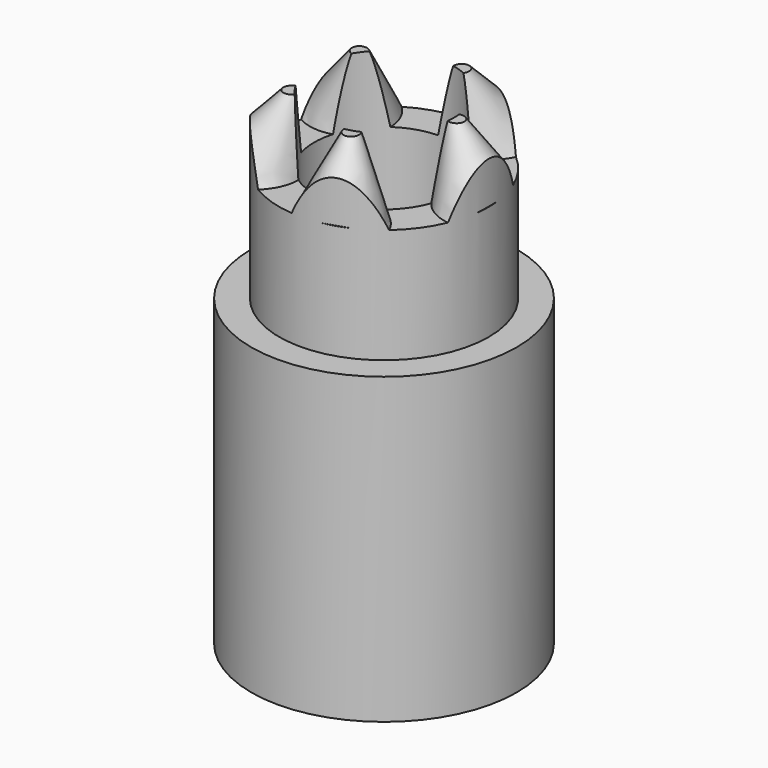
from build123d import *

# Parameters (mm, degrees)
F0_R      = 1.5
F0_R_2    = 1
F1_DEPTH  = 2.6
F5_COUNT  = 5
F5_ANGLE  = 288
F17_DEPTH = 1.64
F0_R_3    = 1.9
F18_DEPTH = 4.35


with BuildPart() as f1:
    # F0 (on Top) → F1 (new body)
    with BuildSketch(Plane.XY):
        Circle(F0_R)
        Circle(F0_R_2, mode=Mode.SUBTRACT)
    extrude(amount=F1_DEPTH)


with BuildPart() as f4:
    # F3 (on Front) → F4 (revolve)
    with BuildSketch(Plane.XZ):
        Polygon((0.9303738137, 2.820600407), (1.375, 1.599), (1.9388155725, 1.804212086), align=None)
    revolve(axis=Axis((1.1526869068, 0, 2.2098002035), (-0.3420201433, 0, 0.9396926208)))


with BuildPart() as f5_1:
    # F5: instance of F4
    add(f4.part.rotate(Axis((0, 0, 0.7995), (0, 0, 1)), 1 * F5_ANGLE / (F5_COUNT - 1)))


with BuildPart() as f5_2:
    # F5: instance of F4
    add(f4.part.rotate(Axis((0, 0, 0.7995), (0, 0, 1)), 2 * F5_ANGLE / (F5_COUNT - 1)))


with BuildPart() as f5_3:
    # F5: instance of F4
    add(f4.part.rotate(Axis((0, 0, 0.7995), (0, 0, 1)), 3 * F5_ANGLE / (F5_COUNT - 1)))


with BuildPart() as f5_4:
    # F5: instance of F4
    add(f4.part.rotate(Axis((0, 0, 0.7995), (0, 0, 1)), 4 * F5_ANGLE / (F5_COUNT - 1)))


with BuildPart() as f6_1:
    # F6: copy of F1
    add(f1.part)


with BuildPart() as f1_1:
    add(f1.part)

    # F7: intersect F4
    add(f4.part, mode=Mode.INTERSECT)



with BuildPart() as f8_1:
    # F8: copy of F6_1
    add(f6_1.part)


with BuildPart() as f9_1:
    # F9: copy of F8_1
    add(f8_1.part)


with BuildPart() as f10_1:
    # F10: copy of F9_1
    add(f9_1.part)


with BuildPart() as f5_1_1:
    add(f5_1.part)

    # F11: intersect F6_1
    add(f6_1.part, mode=Mode.INTERSECT)


with BuildPart() as f5_2_1:
    add(f5_2.part)

    # F12: intersect F8_1
    add(f8_1.part, mode=Mode.INTERSECT)


with BuildPart() as f5_3_1:
    add(f5_3.part)

    # F13: intersect F9_1
    add(f9_1.part, mode=Mode.INTERSECT)


with BuildPart() as f14_1:
    # F14: copy of F10_1
    add(f10_1.part)


with BuildPart() as f10_1_1:
    add(f10_1.part)

    # F15: intersect F5_4
    add(f5_4.part, mode=Mode.INTERSECT)


with BuildPart() as f1_2:
    add(f1_1.part)

    add(f5_1_1.part)  # F17 merges F5_1

    add(f5_2_1.part)  # F17 merges F5_2

    add(f5_3_1.part)  # F17 merges F5_3

    add(f10_1_1.part)  # F17 merges F10_1
    # F0 (on Top) → F17 (join)
    with BuildSketch(Plane.XY):
        Circle(F0_R)
        Circle(F0_R_2, mode=Mode.SUBTRACT)
    extrude(amount=F17_DEPTH)

    # F0 (on Top) → F18 (join)
    with BuildSketch(Plane.XY):
        Circle(F0_R_3)
        Circle(F0_R, mode=Mode.SUBTRACT)
        Circle(F0_R)
        Circle(F0_R_2, mode=Mode.SUBTRACT)
    extrude(amount=-F18_DEPTH)


solid = f1_2.part
